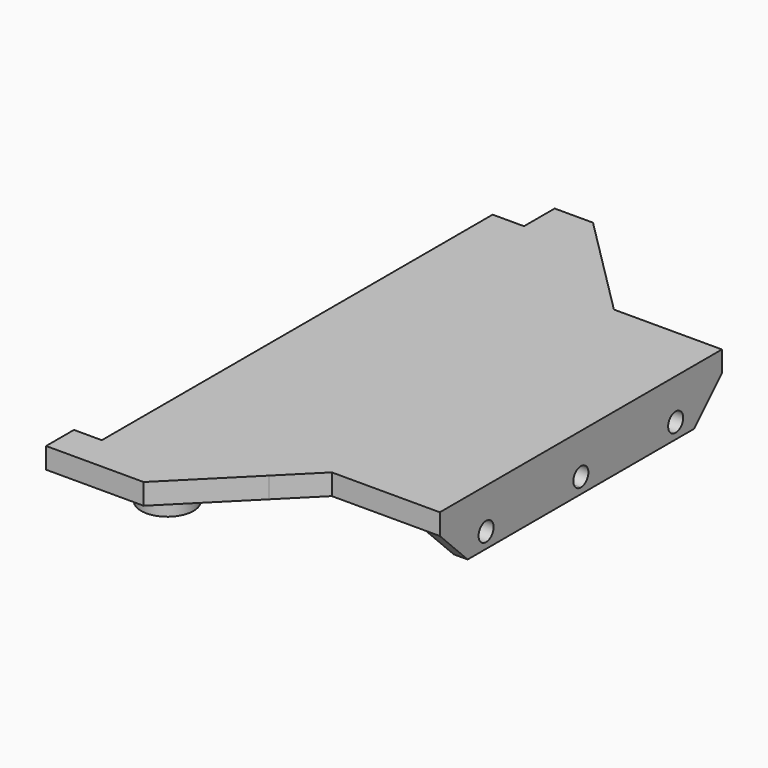
from build123d import *
from build123d import SkipClean  # not in build123d's __all__

# Parameters (mm, degrees)
F0_W                   = 3
F0_H                   = 25.3
F0_W_2                 = 30.5
F1_DEPTH               = 3
F2_DEPTH               = 5
F3_R                   = 1.35
F4_DEPTH               = 500
F7_SIZE                = 5
F8_R                   = 1.35
F9_DEPTH               = 1
F10_W                  = 15
F10_H                  = 15
F11_DEPTH              = 3
F12_W                  = 4
F12_H                  = 5
F13_DEPTH              = 3
F12_W_2                = 4.5
F12_H_2                = 5.5
F14_DEPTH              = 25
F15_DEPTH              = 5
F16_R                  = 3.75
F17_DEPTH              = 2
F20_D                  = 3
F20_DEPTH              = 3
F20_CBORE_D            = 3
F20_CBORE_DEPTH        = 3
F20_TIP                = 0.9012909285
F20_ON_F19_D           = 3
F20_ON_F19_DEPTH       = 3
F20_ON_F19_CBORE_D     = 3
F20_ON_F19_CBORE_DEPTH = 3
F20_ON_F19_TIP         = 0.9012909285
F21_SIZE               = 10
F22_DEPTH              = 1
F23_SIZE               = 4.99999


# Not quite as in the source:
# - a fillet or chamfer is up to 0.001 mm smaller than in the source, because OpenCascade refuses the exact size


with BuildPart() as f1:
    # F0 (on Top) → F1 (new body)
    with BuildSketch(Plane.XY):
        with Locations((16.75, 0)):
            Rectangle(F0_W, F0_H)
        Rectangle(F0_W_2, F0_H)
        with Locations((-16.75, 0)):
            Rectangle(F0_W, F0_H)
    extrude(amount=F1_DEPTH)

    # F0 (on Top) → F2 (join)
    with BuildSketch(Plane.XY):
        with Locations((16.75, 0)):
            Rectangle(F0_W, F0_H)
        with Locations((-16.75, 0)):
            Rectangle(F0_W, F0_H)
    extrude(amount=-F2_DEPTH)

    # F3 (on face) → F4 (cut, symmetric)
    with BuildSketch(Plane(origin=(15.25, 0, 0), x_dir=(0, -1, 0), z_dir=(-1, 0, 0))):
        with BuildLine():
            Line((12.65, -4.15), (12.65, -1.45))
            ThreePointArc((12.65, -1.45), (11.3, -2.8), (12.65, -4.15))
        make_face()
        with Locations((-4.35, -2.8)):
            Circle(F3_R)
    extrude(amount=F4_DEPTH, both=True, mode=Mode.SUBTRACT)

    # F6: F1 across plane


with BuildPart() as f1_1:
    add(f1.part, clean=False)
    with SkipClean():  # cleaning this boolean's faces spoils the solid; the shape is the same uncleaned
        add(f1.part.mirror(Plane.XZ.offset(12.65)), clean=False)

    # F7
    f7_edges = [f1_1.edges().sort_by_distance(p)[0] for p in [
        (-16.75, 12.65, -5),
        (16.75, 12.65, -5),
        (16.75, -37.95, -5),
        (-16.75, -37.95, -5),
    ]]
    chamfer(f7_edges, length=F7_SIZE)

    # F8 (on face) → F9 (cut)
    with BuildSketch(Plane(origin=(-18.25, 0, 0), x_dir=(0, -1, 0), z_dir=(-1, 0, 0))):
        with BuildLine():
            Line((12.65, 0), (-12.65, 0))
            Line((-12.65, 0), (-7.65, -5))
            Line((-7.65, -5), (12.65, -5))
            Line((12.65, -5), (12.65, -4.15))
            ThreePointArc((12.65, -4.15), (11.3, -2.8), (12.65, -1.45))
            Line((12.65, -1.45), (12.65, 0))
        make_face()
        with Locations((-4.35, -2.8)):
            Circle(F8_R, mode=Mode.SUBTRACT)
        with BuildLine():
            Line((37.95, 0), (12.65, 0))
            Line((12.65, 0), (12.65, -1.45))
            ThreePointArc((12.65, -1.45), (14, -2.8), (12.65, -4.15))
            Line((12.65, -4.15), (12.65, -5))
            Line((12.65, -5), (32.95, -5))
            Line((32.95, -5), (37.95, 0))
        make_face()
        with Locations((29.65, -2.8)):
            Circle(F8_R, mode=Mode.SUBTRACT)
    extrude(amount=-F9_DEPTH, mode=Mode.SUBTRACT)

    # F10 (on Top) → F11 (join)
    with BuildSketch(Plane.XY):
        with Locations((-10.75, -45.45)):
            Rectangle(F10_W, F10_H)
        with Locations((-10.75, 20.15)):
            Rectangle(F10_W, F10_H)
    extrude(amount=F11_DEPTH)

    # F12 (on face) → F13 (join)
    with BuildSketch(Plane(origin=(0, 0, 0), x_dir=(1, 0, 0), z_dir=(0, 0, -1))):
        with Locations((-20.25, 50.45)):
            Rectangle(F12_W, F12_H)
    extrude(amount=-F13_DEPTH)

    # F12 (on face) → F14 (cut)
    with BuildSketch(Plane(origin=(0, 0, 0), x_dir=(1, 0, 0), z_dir=(0, 0, -1))):
        with Locations((-16, -24.9)):
            Rectangle(F12_W_2, F12_H_2)
    extrude(amount=-F14_DEPTH, mode=Mode.SUBTRACT)

    # F15 (add): faces of the model
    f15_faces = [f1_1.faces().sort_by_distance(p)[0] for p in [
        (-18.25, 0, 1.5),
        (-18.25, -25.3, 1.5),
        (-18.25, -42.95, 1.5),
        (-18.25, 17.4, 1.5),
        (-22.25, -50.45, 1.5),
        (-13.75, 24.9, 1.5),
    ]]
    extrude(f15_faces, amount=F15_DEPTH)

    # F16 (on face) → F17 (join)
    with BuildSketch(Plane(origin=(0, 0, 0), x_dir=(1, 0, 0), z_dir=(0, 0, -1))):
        with BuildLine():
            Line((-13.75, -22.15), (-18, -22.15))
            ThreePointArc((-18, -22.15), (-16.7185522073, -24.9728974477), (-13.75, -25.8665171868))
            Line((-13.75, -25.8665171868), (-13.75, -22.15))
        make_face()
        with BuildLine():
            ThreePointArc((-13.75, -25.8665171868), (-11.4271025523, -24.6185522073), (-10.5, -22.15))
            ThreePointArc((-10.5, -22.15), (-14.25, -18.4), (-18, -22.15))
            Line((-18, -22.15), (-13.75, -22.15))
            Line((-13.75, -22.15), (-13.75, -25.8665171868))
        make_face()
        with Locations((-14.25, 47.45)):
            Circle(F16_R)
    extrude(amount=F17_DEPTH)

    # F20
    with Locations(Plane(origin=(0, 0, -2), x_dir=(1, 0, 0), z_dir=(0, 0, -1))):
        with Locations((-14.25, 47.45)):
            CounterBoreHole(F20_D / 2, F20_CBORE_D / 2, F20_CBORE_DEPTH, depth=F20_DEPTH)
            with Locations((0, 0, -(F20_DEPTH + F20_TIP / 2))):  # 118° drill point
                Cone(0, F20_D / 2, F20_TIP, mode=Mode.SUBTRACT)

    # F20 on F19
    with Locations(Plane(origin=(0, 0, -2), x_dir=(1, 0, 0), z_dir=(0, 0, -1))):
        with Locations((-14.25, -22.15)):
            CounterBoreHole(F20_ON_F19_D / 2, F20_ON_F19_CBORE_D / 2, F20_ON_F19_CBORE_DEPTH, depth=F20_ON_F19_DEPTH)
            with Locations((0, 0, -(F20_ON_F19_DEPTH + F20_ON_F19_TIP / 2))):  # 118° drill point
                Cone(0, F20_ON_F19_D / 2, F20_ON_F19_TIP, mode=Mode.SUBTRACT)

    # F21
    f21_edges = [f1_1.edges().sort_by_distance(p)[0] for p in [
        (-3.25, 27.65, 1.5),
        (-3.25, -52.95, 1.5),
    ]]
    chamfer(f21_edges, length=F21_SIZE)

    # F22 (cut): a face of the model
    f22_faces = [f1_1.faces().sort_by_distance(p)[0] for p in [
        (18.25, -12.65, -0.7538732148),
    ]]
    extrude(f22_faces, amount=-F22_DEPTH, mode=Mode.SUBTRACT)

    # F23 (size 5 in the source; OpenCascade refuses exactly that, so slightly less here)
    f23_edges = [f1_1.edges().sort_by_distance(p)[0] for p in [
        (-3.25, -37.95, 1.5),
        (-3.25, 12.65, 1.5),
    ]]
    chamfer(f23_edges, length=F23_SIZE)


solid = f1_1.part
